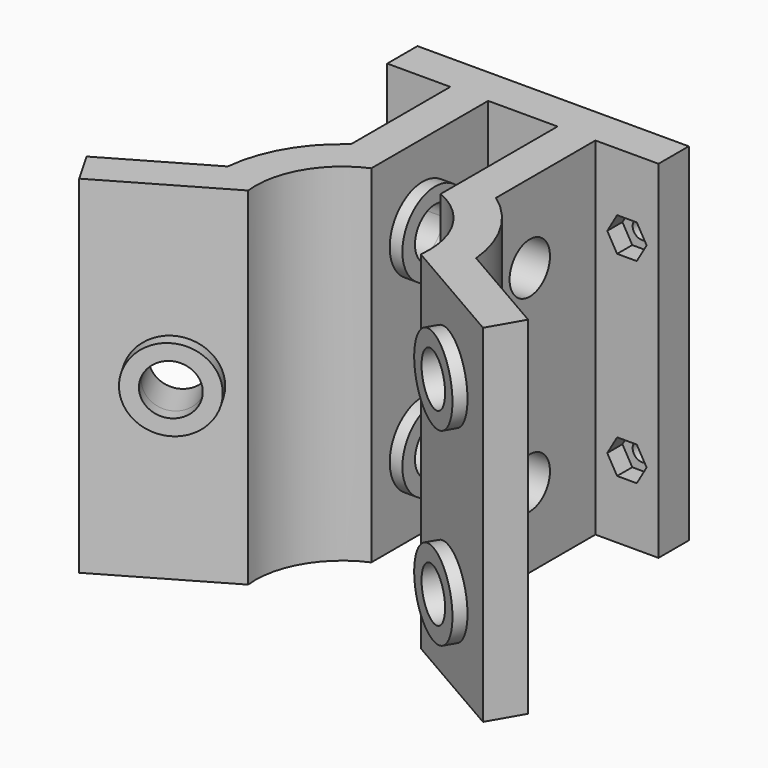
from build123d import *

# Parameters (mm, degrees)
F8_W             = 10
F8_H             = 6
F9_DEPTH         = 55
F10_R            = 11
F10_R_2          = 4
F11_DEPTH        = 7
F12_R            = 6.5
F16_DEPTH        = 2
F17_D            = 8
F17_ON_F12_D     = 8
F17_ON_F12_DEPTH = 48.1792152495
F17_ON_F14_D     = 8
F17_ON_F14_DEPTH = 29.5010080128
F17_ON_F15_D     = 8
F17_ON_F15_DEPTH = 29.5010080128
F13_R            = 6.5
F18_DEPTH        = 2
F15_R            = 6.5
F19_DEPTH        = 2
F14_R            = 6.5
F20_DEPTH        = 2
F21_D            = 8
F21_ON_F15_D     = 8
F21_ON_F13_D     = 8
F23_D            = 3
F23_DEPTH        = 6
F23_TIP          = 0.9012909285
F24_R            = 1.5
F25_DEPTH        = 3


# Not quite as in the source:
# - a feature names something its author has since deleted; it is built from what else it names


with BuildPart() as f9:
    # F8 (on Top) → F9 (new body)
    with BuildSketch(Plane.XY):
        with BuildLine():
            ThreePointArc((-13.687342856, -1.5515381213), (-11.9294999371, 6.8875), (-5.5, 12.6293556843))
            Line((-5.5, 12.6293556843), (-5.5, 35.775))
            Line((-5.5, 35.775), (5.5, 35.775))
            Line((5.5, 35.775), (5.5, 12.6293556843))
            ThreePointArc((5.5, 12.6293556843), (11.9294999371, 6.8875), (13.687342856, -1.5515381213))
            Line((13.687342856, -1.5515381213), (32.0000080128, -12.1243602792))
            Line((32.0000080128, -12.1243602792), (35.0000080128, -6.9282078565))
            Line((35.0000080128, -6.9282078565), (19.6819944283, 1.91565141))
            ThreePointArc((19.6819944283, 1.91565141), (17.1256523598, 9.8875), (11.5, 16.087281467))
            Line((11.5, 16.087281467), (11.5, 35.775))
            Line((11.5, 35.775), (11.5, 41.775))
            Line((11.5, 41.775), (-11.5, 41.775))
            Line((-11.5, 41.775), (-11.5, 35.775))
            Line((-11.5, 35.775), (-11.5, 16.087281467))
            ThreePointArc((-11.5, 16.087281467), (-17.1256523598, 9.8875), (-19.6819944283, 1.91565141))
            Line((-19.6819944283, 1.91565141), (-35.0000080128, -6.9282078565))
            Line((-35.0000080128, -6.9282078565), (-32.0000080128, -12.1243602792))
            Line((-32.0000080128, -12.1243602792), (-13.687342856, -1.5515381213))
        make_face()
        with Locations((-16.5, 38.775)):
            Rectangle(F8_W, F8_H)
        with Locations((16.5, 38.775)):
            Rectangle(F8_W, F8_H)
    extrude(amount=F9_DEPTH)

    # F12 (on face) → F16 (join)
    with BuildSketch(Plane(origin=(-2.75, 4.7631397208, 0), x_dir=(0.8660254038, 0.5, 0), z_dir=(0.5, -0.8660254038, 0))):
        with Locations((-22, 27.5)):
            Circle(F12_R)
    extrude(amount=F16_DEPTH)

    # F17 (through all)
    with Locations(Plane(origin=(2.75, 4.7631397208, 0), x_dir=(0.8660254038, -0.5, 0), z_dir=(-0.5, -0.8660254038, 0))):
        with Locations((22, 42.5), (22, 12.5)):
            Hole(F17_D / 2)

    # F17 on F12 (through all, one way)
    with BuildSketch(Plane(origin=(-2.75, 4.7631397208, 0), x_dir=(0.8660254038, 0.5, 0), z_dir=(0.5, -0.8660254038, 0))):
        with Locations((-22, 27.5)):
            Circle(F17_ON_F12_D / 2)
    extrude(amount=-F17_ON_F12_DEPTH, mode=Mode.SUBTRACT)

    # F17 on F14 (through all, one way)
    with BuildSketch(Plane(origin=(5.5, 0, 0), x_dir=(0, -1, 0), z_dir=(-1, 0, 0))):
        with Locations((-22.775, 42.5), (-22.775, 12.5)):
            Circle(F17_ON_F14_D / 2)
    extrude(amount=-F17_ON_F14_DEPTH, mode=Mode.SUBTRACT)

    # F17 on F15 (through all, one way)
    with BuildSketch(Plane.YZ.offset(-5.5)):
        with Locations((22.775, 42.5), (22.775, 12.5)):
            Circle(F17_ON_F15_D / 2)
    extrude(amount=-F17_ON_F15_DEPTH, mode=Mode.SUBTRACT)

    # F13 (on face) → F18 (join)
    with BuildSketch(Plane(origin=(2.75, 4.7631397208, 0), x_dir=(0.8660254038, -0.5, 0), z_dir=(-0.5, -0.8660254038, 0))):
        with Locations((22, 12.5)):
            Circle(F13_R)
        with Locations((22, 42.5)):
            Circle(F13_R)
    extrude(amount=F18_DEPTH)

    # F15 (on face) → F19 (join)
    with BuildSketch(Plane.YZ.offset(-5.5)):
        with Locations((22.775, 12.5)):
            Circle(F15_R)
        with Locations((22.775, 42.5)):
            Circle(F15_R)
    extrude(amount=F19_DEPTH)

    # F14 (on face) → F20 (join)
    with BuildSketch(Plane(origin=(5.5, 0, 0), x_dir=(0, -1, 0), z_dir=(-1, 0, 0))):
        with Locations((-22.775, 12.5)):
            Circle(F14_R)
        with Locations((-22.775, 42.5)):
            Circle(F14_R)
    extrude(amount=F20_DEPTH)

    # F21 (through all)
    with Locations(Plane(origin=(-2.75, 4.7631397208, 0), x_dir=(0.8660254038, 0.5, 0), z_dir=(-0.5, 0.8660254038, 0))):
        with Locations((-22, -27.5)):
            Hole(F21_D / 2)

    # F21 on F15 (through all)
    with Locations(Plane(origin=(-5.5, 0, 0), x_dir=(0, 1, 0), z_dir=(-1, 0, 0))):
        with Locations((22.775, -42.5), (22.775, -12.5)):
            Hole(F21_ON_F15_D / 2)

    # F21 on F13 (through all)
    with Locations(Plane(origin=(2.75, 4.7631397208, 0), x_dir=(0.8660254038, -0.5, 0), z_dir=(0.5, 0.8660254038, 0))):
        with Locations((22, -42.5), (22, -12.5)):
            Hole(F21_ON_F13_D / 2)

    # F23
    with Locations(Plane(origin=(0, 41.775, 0), x_dir=(-1, 0, 0), z_dir=(0, 1, 0))):
        with Locations((16.5, 12), (-16.5, 12), (-16.5, 43), (16.5, 43)):
            Hole(F23_D / 2, depth=F23_DEPTH)
            with Locations((0, 0, -(F23_DEPTH + F23_TIP / 2))):  # 118° drill point
                Cone(0, F23_D / 2, F23_TIP, mode=Mode.SUBTRACT)

    # F24 (on face) → F25 (cut)
    with BuildSketch(Plane.XZ.offset(-35.775)):
        Polygon((-18.0588457268, 9.3), (-14.9411542732, 9.3), (-13.3823085464, 12), (-14.9411542732, 14.7), (-18.0588457268, 14.7), (-19.6176914536, 12), align=None)
        Polygon((-14.9411542732, 45.7), (-18.0588457268, 45.7), (-19.6176914536, 43), (-18.0588457268, 40.3), (-14.9411542732, 40.3), (-13.3823085464, 43), align=None)
        Polygon((18.0588457268, 14.7), (14.9411542732, 14.7), (13.3823085464, 12), (14.9411542732, 9.3), (18.0588457268, 9.3), (19.6176914536, 12), align=None)
        with Locations((16.5, 12)):
            Circle(F24_R, mode=Mode.SUBTRACT)
        Polygon((18.0588457268, 45.7), (14.9411542732, 45.7), (13.3823085464, 43), (14.9411542732, 40.3), (18.0588457268, 40.3), (19.6176914536, 43), align=None)
        with Locations((16.5, 43)):
            Circle(F24_R, mode=Mode.SUBTRACT)
    extrude(amount=-F25_DEPTH, mode=Mode.SUBTRACT)


with BuildPart() as f11:
    # F10 (on Top) → F11 (new body)
    with BuildSketch(Plane.XY):
        with Locations((-55.1071129739, 58.1275820732)):
            Circle(F10_R)
        with Locations((-55.1071129739, 58.1275820732)):
            Circle(F10_R_2, mode=Mode.SUBTRACT)
    extrude(amount=F11_DEPTH)


solid = Compound([f9.part, f11.part])
